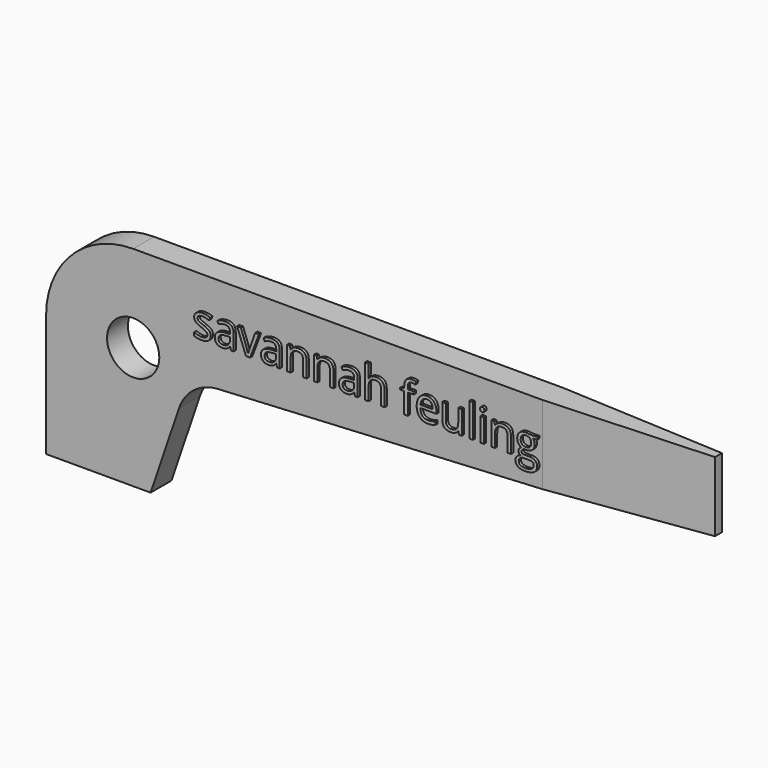
from build123d import *

# Parameters (mm, degrees)
F1_DEPTH     = 2.38125
F2_R         = 2.38125
F3_DEPTH     = 2.38225
F5_DEPTH     = 25.4
F6_TEXT_SIZE = 3.9839231448
F7_DEPTH     = 0.254


# Not quite as in the source:
# - Text() gives the source's letters only with a copy of the font that has no kerning and outlines rounded to 1/6400 em; it was checked with that copy


with BuildPart() as f1:
    # F0 (on Front) → F1 (new body)
    with BuildSketch(Plane.XZ):
        with BuildLine():
            Line((60.325, 19.05), (7.9375, 19.05))
            ThreePointArc((7.9375, 19.05), (2.3248399243, 16.7251600757), (0, 11.1125))
            Line((0, 11.1125), (0, 0))
            Line((0, 0), (9.525, 0))
            Line((9.525, 0), (12.1173647876, 7.6271664624))
            ThreePointArc((12.1173647876, 7.6271664624), (13.4786145605, 9.5135918491), (15.6631963617, 10.3130942181))
            Line((15.6631963617, 10.3130942181), (60.325, 12.7))
            Line((60.325, 12.7), (60.325, 19.05))
        make_face()
    extrude(amount=F1_DEPTH)

    # F2 (on face) → F3 (cut, through all)
    with BuildSketch(Plane.XZ.offset(2.38125)):
        with Locations((7.9375, 11.1125)):
            Circle(F2_R)
    extrude(amount=-F3_DEPTH, mode=Mode.SUBTRACT)

    # F4 (on face) → F5 (cut)
    with BuildSketch(Plane.XY.offset(19.05)):
        Polygon((60.325, -2.38125), (60.325, -1.5875), (45.24375, -2.38125), align=None)
        Polygon((60.325, 0), (45.24375, 0), (60.325, -0.79375), align=None)
    extrude(amount=-F5_DEPTH, mode=Mode.SUBTRACT)

    # F6 (on face) → F7 (join)
    with BuildSketch(Plane.XZ.offset(2.38125)):
        with Locations((13.49375, 13.9545001732)):
            Text('savannah feuling', F6_TEXT_SIZE, font='Open Sans', text_align=(TextAlign.LEFT, TextAlign.BOTTOM))
    extrude(amount=F7_DEPTH)


solid = f1.part
